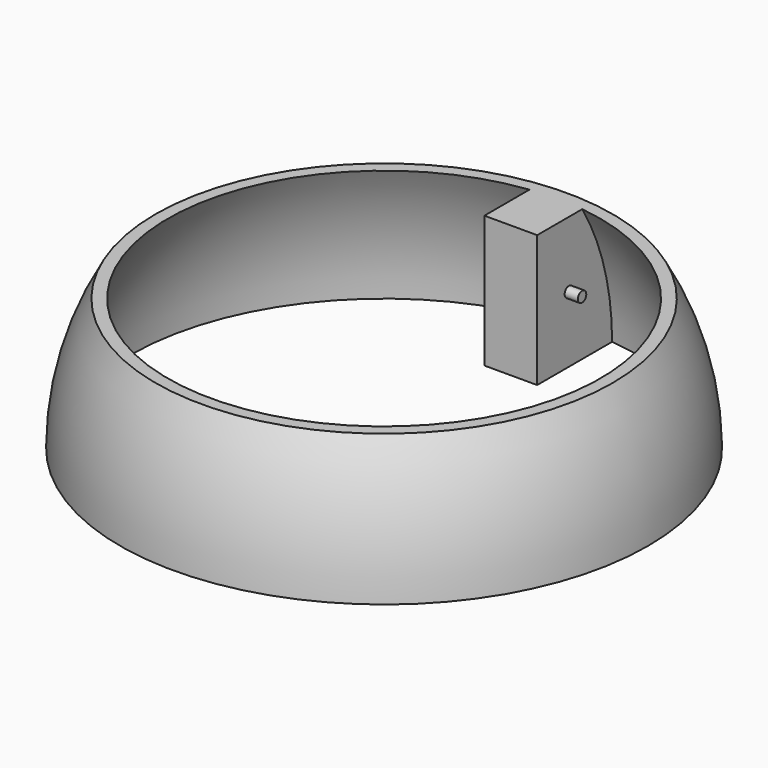
from build123d import *

# Parameters (mm, degrees)
F2_T     = -4
F4_W     = 20
F4_H     = 50
F5_REACH = 93.8526480713
F6_R     = 2
F7_DEPTH = 5


with BuildPart() as f1:
    # F0 (on Front) → F1 (revolve)
    with BuildSketch(Plane.XZ):
        with BuildLine():
            Line((0, 0), (100, 0))
            ThreePointArc((100, 0), (96.5925826289, 25.8819045103), (86.6025403784, 50))
            Line((86.6025403784, 50), (0, 50))
            Line((0, 50), (0, 0))
        make_face()
    revolve(axis=Axis((0, 0, 53.0949570239), (0, 0, 1)))

    # F2
    f2_openings = [f1.faces().sort_by_distance(p)[0] for p in [
        (0, 0, 0),
        (0, 0, 50),
    ]]
    offset(amount=F2_T, openings=f2_openings)

    f5_end = f1.faces().sort_by_distance((-96.5925826289, 0, 25.8819045103))[0]
    # F4 (on offset) → F5 (join, up to a face of the model that its end follows)
    with BuildSketch(Plane.XZ.offset(-60)):
        with Locations((0, 25)):
            Rectangle(F4_W, F4_H)
    f5_long = extrude(amount=-F5_REACH, mode=Mode.PRIVATE)
    add(split(f5_long, bisect_by=f5_end, keep=Keep.BOTTOM, mode=Mode.PRIVATE))

    # F6 (on face) → F7 (join)
    with BuildSketch(Plane.YZ.offset(10)):
        with Locations((75, 25)):
            Circle(F6_R)
    extrude(amount=F7_DEPTH)


solid = f1.part
